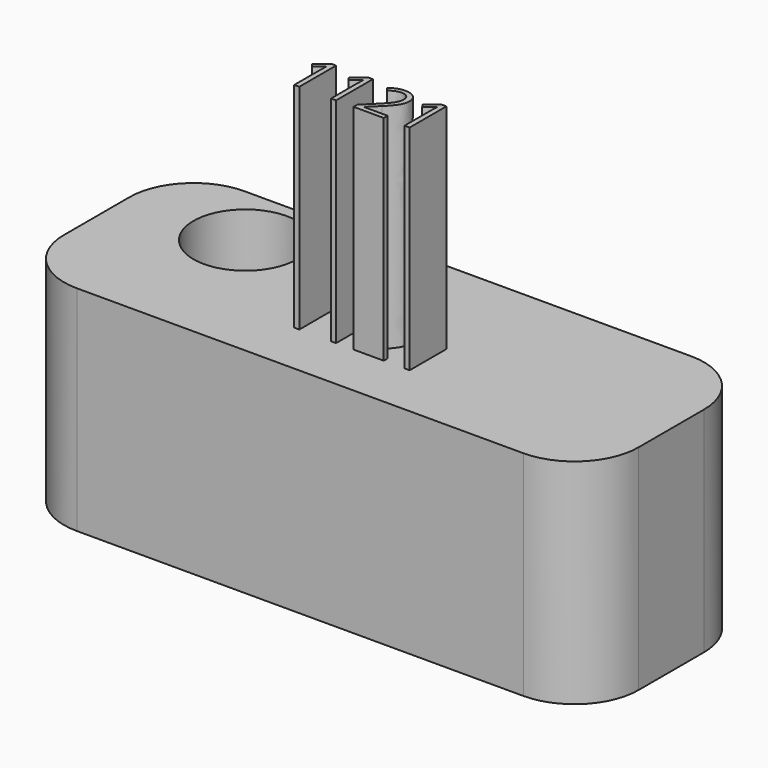
from build123d import *

# Parameters (mm, degrees)
F0_R         = 6.1669790196
F1_DEPTH     = 25.4
F2_TEXT_SIZE = 7.6446889175
F3_DEPTH     = 25.4


# Not quite as in the source:
# - Text() gives the source's letters only with a copy of the font that has no kerning and outlines rounded to 1/6400 em; it was checked with that copy


with BuildPart() as f1:
    # F0 (on Top) → F1 (new body)
    with BuildSketch(Plane.XY):
        with BuildLine():
            ThreePointArc((0, 26.1999064136), (-2.2318463274, 31.5880600862), (-7.62, 33.8199064136))
            Line((-7.62, 33.8199064136), (-60.68483675, 33.8199064136))
            ThreePointArc((-60.68483675, 33.8199064136), (-66.0729904227, 31.5880600862), (-68.30483675, 26.1999064136))
            Line((-68.30483675, 26.1999064136), (-68.30483675, 16.4876586747))
            ThreePointArc((-68.30483675, 16.4876586747), (-66.0729904227, 11.0995050021), (-60.68483675, 8.8676586747))
            Line((-60.68483675, 8.8676586747), (-7.62, 8.8676586747))
            ThreePointArc((-7.62, 8.8676586747), (-2.2318463274, 11.0995050021), (0, 16.4876586747))
            Line((0, 16.4876586747), (0, 26.1999064136))
        make_face()
        with Locations((-54.5178577304, 26.1999064136)):
            Circle(F0_R, mode=Mode.SUBTRACT)
    extrude(amount=F1_DEPTH)

    # F2 (on face) → F3 (join)
    with BuildSketch(Plane.XY.offset(25.4)):
        with Locations((-42.041733861, 15.2891874313)):
            Text('1121', F2_TEXT_SIZE, font='Open Sans', text_align=(TextAlign.LEFT, TextAlign.BOTTOM))
    extrude(amount=F3_DEPTH)


solid = f1.part
